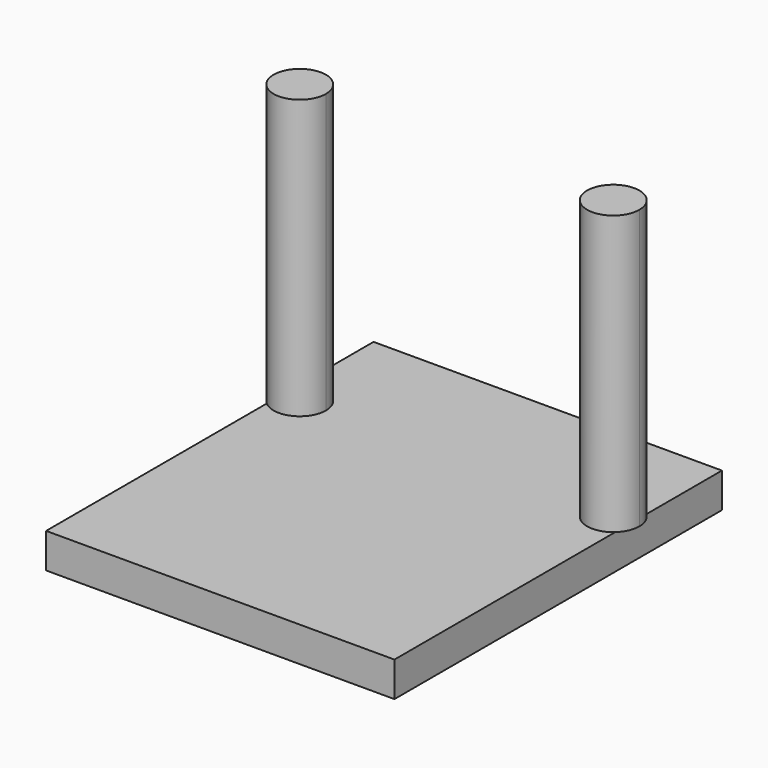
from build123d import *

# Parameters (mm, degrees)
F1_DEPTH = 203.2
F2_R     = 3.9466394405
F3_DEPTH = 25.4


# Not quite as in the source:
# - the program builds the solid bodies; features that only make, move or delete a surface that nothing else refers to are left out


with BuildPart() as f1:
    # F0 (on Top) → F1 (new body)
    with BuildSketch(Plane.XY):
        with BuildLine():
            ThreePointArc((175.5912042022, 11.5693333262), (163.3386650124, 29.3653167645), (142.3421725451, 24.2693333262))
            ThreePointArc((142.3421725451, 24.2693333262), (149.743743392, -6.226650112), (175.5912042022, 11.5693333262))
        make_face()
    extrude(amount=F1_DEPTH)


with BuildPart() as f1b:
    # F0 (on Top) → F1, piece 2 (new body)
    with BuildSketch(Plane.XY):
        with BuildLine():
            ThreePointArc((-53.0087957978, 11.5693333262), (-54.2628123596, 18.3667941364), (-57.8597641407, 24.2693333262))
            ThreePointArc((-57.8597641407, 24.2693333262), (-89.8547792361, 4.771872516), (-53.0087957978, 11.5693333262))
        make_face()
    extrude(amount=F1_DEPTH)


with BuildPart() as f3:
    # F2 (on Top) → F3 (new body)
    with BuildSketch(Plane.XY):
        Polygon((169.2891323054, -203.8045942991), (169.2891323054, 18.4454057009), (169.2891323054, 94.6454057009), (37.2091323054, 94.6454057009), (-84.7108676946, 94.6454057009), (-84.7108676946, 18.4454057009), (-84.7108676946, -203.8045942991), align=None)
        with Locations((42.2891323054, 0)):
            Circle(F2_R, mode=Mode.SUBTRACT)
        with Locations((42.2891323054, 0)):
            Circle(F2_R)
    extrude(amount=-F3_DEPTH)


solid = Compound([f1.part, f1b.part, f3.part])
